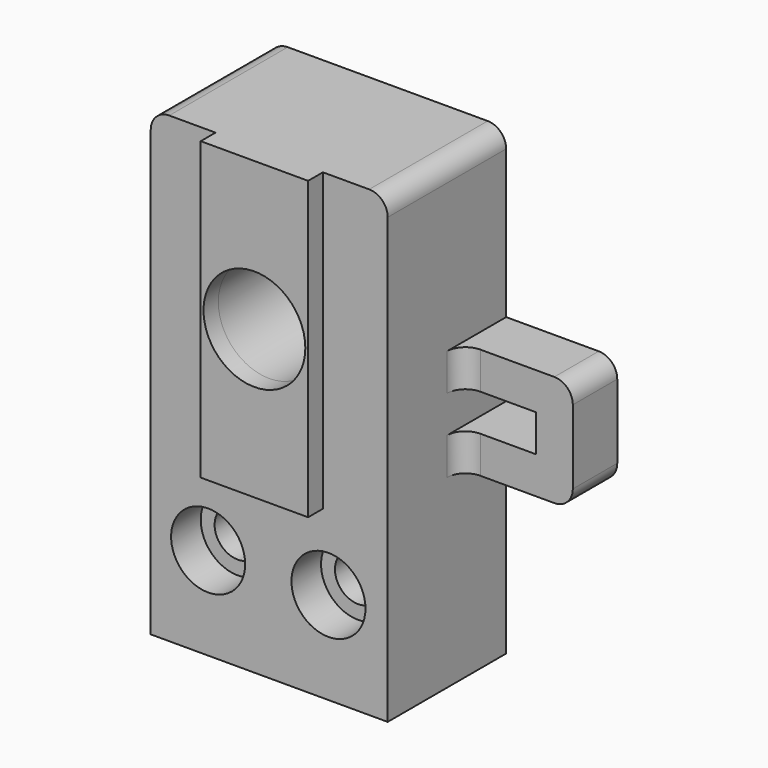
from build123d import *
from build123d import SkipClean  # not in build123d's __all__

# Parameters (mm, degrees)
F1_W          = 12.8
F1_H          = 25
F1_R          = 1.25
F2_DEPTH      = 8
F3_R          = 2.75
F4_DEPTH      = 8.001
F5_R          = 2
F6_DEPTH      = 2
F7_R          = 2.75
F8_DEPTH      = 1
F9_W          = 3
F9_H          = 6
F10_DEPTH     = 6
F11_W         = 4
F11_H         = 2
F12_DEPTH     = 3
F13_T1_DEPTH  = 2
F13_T3_DEPTH  = 2
F13_T8_DEPTH  = 4.5
F13_T13_DEPTH = 4.5
F13_T15_DEPTH = 8
F13_T17_DEPTH = 13
F14_R         = 4.5
F15_DEPTH     = 3


# Not quite as in the source:
# - a fillet or chamfer that OpenCascade refuses, or shapes differently, is made with other operations: its cross-section is extruded or revolved along the edge and cut away or added
# - after a boolean that leaves OpenCascade's solid faulty, fix() repairs it


with BuildPart() as f2:
    # F1 (on Front) → F2 (new body)
    with BuildSketch(Plane.XZ):
        with Locations((0, 9.25)):
            Rectangle(F1_W, F1_H)
        with Locations((-3.3, 1.75)):
            Circle(F1_R, mode=Mode.SUBTRACT)
        with Locations((3.2, 1.75)):
            Circle(F1_R, mode=Mode.SUBTRACT)
    extrude(amount=F2_DEPTH)

    # F3 (on face) → F4 (cut, through all)
    with BuildSketch(Plane(origin=(0, 0, 0), x_dir=(-1, 0, 0), z_dir=(0, 1, 0))):
        with Locations((0, 13.75)):
            Circle(F3_R)
    extrude(amount=-F4_DEPTH, mode=Mode.SUBTRACT)

    # F5 (on face) → F6 (cut)
    with BuildSketch(Plane.XZ.offset(8)):
        with Locations((-3.3, 1.75)):
            Circle(F5_R)
        with Locations((3.2, 1.75)):
            Circle(F5_R)
    extrude(amount=-F6_DEPTH, mode=Mode.SUBTRACT)

    # F7 (on face) → F8 (join)
    with BuildSketch(Plane.XZ.offset(8)):
        Polygon((-2.9, 5.75), (0, 5.75), (2.9, 5.75), (2.9, 21.75), (0, 21.75), (-2.9, 21.75), align=None)
        with Locations((0, 13.75)):
            Circle(F7_R, mode=Mode.SUBTRACT)
    with SkipClean():  # cleaning this boolean's faces spoils the solid; the shape is the same uncleaned
        extrude(amount=F8_DEPTH)

    # F9 (on face) → F10 (join)
    with BuildSketch(Plane.YZ.offset(6.4)):
        with Locations((-1.5, 9.75)):
            Rectangle(F9_W, F9_H)
    extrude(amount=F10_DEPTH)

    add(f2.part.fix(), mode=Mode.REPLACE)

    # F11 (on face) → F12 (cut, through all)
    with BuildSketch(Plane(origin=(0, 0, 0), x_dir=(-1, 0, 0), z_dir=(0, 1, 0))):
        with Locations((-8.4, 9.75)):
            Rectangle(F11_W, F11_H)
    extrude(amount=-F12_DEPTH, mode=Mode.SUBTRACT)

    add(f2.part.fix(), mode=Mode.REPLACE)

    # F13: fillet of radius 1 on 6 edges, made by hand

    # F13_s2 → F13_t1 (join)
    with BuildSketch(Plane.XY.offset(10.75)):
        with BuildLine():
            ThreePointArc((6.4, -4), (6.6928932188, -3.2928932188), (7.4, -3))
            Line((7.4, -3), (6.4, -3))
            Line((6.4, -3), (6.4, -4))
        make_face()
    extrude(amount=F13_T1_DEPTH)

    # F13_s4 → F13_t3 (join)
    with BuildSketch(Plane.XY.offset(6.75)):
        with BuildLine():
            ThreePointArc((6.4, -4), (6.6928932188, -3.2928932188), (7.4, -3))
            Line((7.4, -3), (6.4, -3))
            Line((6.4, -3), (6.4, -4))
        make_face()
    extrude(amount=F13_T3_DEPTH)


with BuildPart() as f13_tool6:
    # F13_s7 → F13_t8 (new body)
    with BuildSketch(Plane.XY.offset(12.75)):
        with BuildLine():
            ThreePointArc((6.4, -4), (6.6928932188, -3.2928932188), (7.4, -3))
            Line((7.4, -3), (6.4, -3))
            Line((6.4, -3), (6.4, -4))
        make_face()
    extrude(amount=-F13_T8_DEPTH)

    split(bisect_by=Plane.XY.offset(8.75), keep=Keep.BOTTOM)


with BuildPart() as f2_1:
    add(f2.part, clean=False)

    # F13_t5: union F13_tool6
    add(f13_tool6.part)


with BuildPart() as f13_tool11:
    # F13_s12 → F13_t13 (new body)
    with BuildSketch(Plane.XY.offset(11.25)):
        with BuildLine():
            ThreePointArc((6.4, -4), (6.6928932188, -3.2928932188), (7.4, -3))
            Line((7.4, -3), (6.4, -3))
            Line((6.4, -3), (6.4, -4))
        make_face()
    extrude(amount=-F13_T13_DEPTH)

    split(bisect_by=Plane.XY.offset(10.75), keep=Keep.TOP)


with BuildPart() as f2_2:
    add(f2_1.part, clean=False)

    # F13_t10: union F13_tool11
    add(f13_tool11.part)

    # F13_s16 → F13_t15 (cut)
    with BuildSketch(Plane.XZ.offset(-2.5)):
        with BuildLine():
            ThreePointArc((11.4, 6.75), (12.1071067812, 7.0428932188), (12.4, 7.75))
            Line((12.4, 7.75), (12.4, 6.75))
            Line((12.4, 6.75), (11.4, 6.75))
        make_face()
        with BuildLine():
            ThreePointArc((11.4, 12.75), (12.1071067812, 12.4571067812), (12.4, 11.75))
            Line((12.4, 11.75), (12.4, 12.75))
            Line((12.4, 12.75), (11.4, 12.75))
        make_face()
    extrude(amount=F13_T15_DEPTH, mode=Mode.SUBTRACT)

    # F13_s18 → F13_t17 (cut)
    with BuildSketch(Plane.XZ.offset(-2.5)):
        with BuildLine():
            ThreePointArc((5.4, 21.75), (6.1071067812, 21.4571067812), (6.4, 20.75))
            Line((6.4, 20.75), (6.4, 21.75))
            Line((6.4, 21.75), (5.4, 21.75))
        make_face()
        with BuildLine():
            ThreePointArc((-5.4, 21.75), (-6.1071067812, 21.4571067812), (-6.4, 20.75))
            Line((-6.4, 20.75), (-6.4, 21.75))
            Line((-6.4, 21.75), (-5.4, 21.75))
        make_face()
    extrude(amount=F13_T17_DEPTH, mode=Mode.SUBTRACT)

    # F14 (on face) → F15 (cut)
    with BuildSketch(Plane(origin=(0, 0, 0), x_dir=(-1, 0, 0), z_dir=(0, 1, 0))):
        with Locations((0, 13.75)):
            Circle(F14_R)
    extrude(amount=-F15_DEPTH, mode=Mode.SUBTRACT)


solid = f2_2.part
